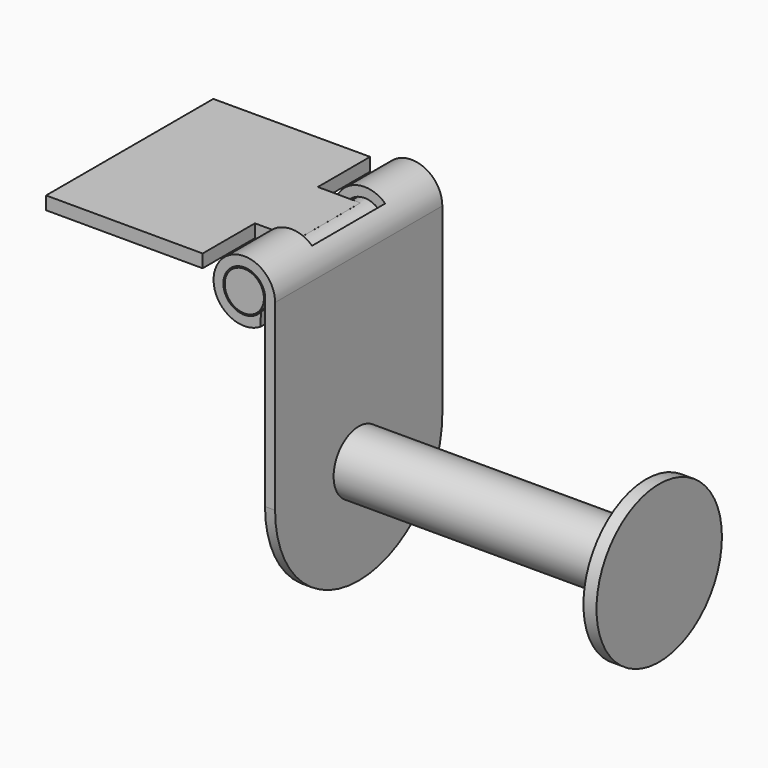
from build123d import *

# Parameters (mm, degrees)
F1_DEPTH  = 20.32
F2_W      = 6.6402247176
F2_H      = 4.445
F3_DEPTH  = 50.8
F4_R      = 1.905
F5_DEPTH  = 20.32
F8_DEPTH  = 1.27
F9_R      = 10.15999
F10_R     = 3.048
F11_DEPTH = 27.94
F12_R     = 7.62
F13_DEPTH = 1.27


# Not quite as in the source:
# - a fillet or chamfer is up to 0.001 mm smaller than in the source, because OpenCascade refuses the exact size


with BuildPart() as f1:
    # F0 (on Front) → F1 (new body)
    with BuildSketch(Plane.XZ):
        with BuildLine():
            Line((0, 28.2609894363), (0, 0))
            Line((0, 0), (0.9779490576, 0))
            Line((0.9779490576, 0), (0.9779490576, 27.94))
            ThreePointArc((0.9779490576, 27.94), (-4.6212260032, 29.4002809847), (-0.4484143049, 25.3914377043))
            Line((-0.4484143049, 25.3914377043), (-0.3938082239, 26.7019847298))
            ThreePointArc((-0.3938082239, 26.7019847298), (-3.9875154003, 28.439004333), (0, 28.2609894363))
        make_face()
    extrude(amount=F1_DEPTH)

    # F2 (on face) → F3 (cut)
    with BuildSketch(Plane(origin=(0, 0, 0), x_dir=(1, 0, 0), z_dir=(0, 0, -1))):
        with Locations((-3.3201123588, 7.9375)):
            Rectangle(F2_W, F2_H)
        with Locations((-3.3201123588, 12.3825)):
            Rectangle(F2_W, F2_H)
        Polygon((-6.6402247176, 5.715), (-6.6402247176, 10.16), (-6.6402247176, 14.605), (-8.3473562263, 14.605), (-8.3473562263, 5.715), align=None)
    extrude(amount=-F3_DEPTH, mode=Mode.SUBTRACT)

    # F9 (radius 10.16 in the source; OpenCascade refuses exactly that, so slightly less here)
    f9_edges = [f1.edges().sort_by_distance(p)[0] for p in [
        (0.488975, 0, 0),
        (0.488975, -20.32, 0),
    ]]
    fillet(f9_edges, radius=F9_R)

    # F10 (on face) → F11 (join)
    with BuildSketch(Plane.YZ.offset(0.9779490576)):
        with Locations((-10.16, 10.16)):
            Circle(F10_R)
    extrude(amount=F11_DEPTH)

    # F12 (on face) → F13 (join)
    with BuildSketch(Plane.YZ.offset(28.9179490576)):
        with Locations((-10.16, 10.16)):
            Circle(F12_R)
    extrude(amount=F13_DEPTH)


with BuildPart() as f5:
    # F4 (on face) → F5 (new body)
    with BuildSketch(Plane.XZ.offset(20.32)):
        with Locations((-2.0120612164, 27.94)):
            Circle(F4_R)
    extrude(amount=-F5_DEPTH)

    # F7 (on offset) → F8 (join)
    with BuildSketch(Plane.XY.offset(28.575)):
        Polygon((-6.0613232421, -6.325361908), (-6.0613478435, -13.9727453345), (-1.9049090762, -13.9727453345), (-1.9049980218, -10.1627453355), (-1.9049980218, -6.3527453355), align=None)
        Polygon((-6.0613478435, -20.3227453345), (-6.0613478435, -13.9727453345), (-6.0613232421, -6.325361908), (-6.0613232421, 0.024638092), (-21.3013232421, 0.024638092), (-21.3013232421, -20.295361908), align=None)
    extrude(amount=F8_DEPTH)


solid = Compound([f1.part, f5.part])
